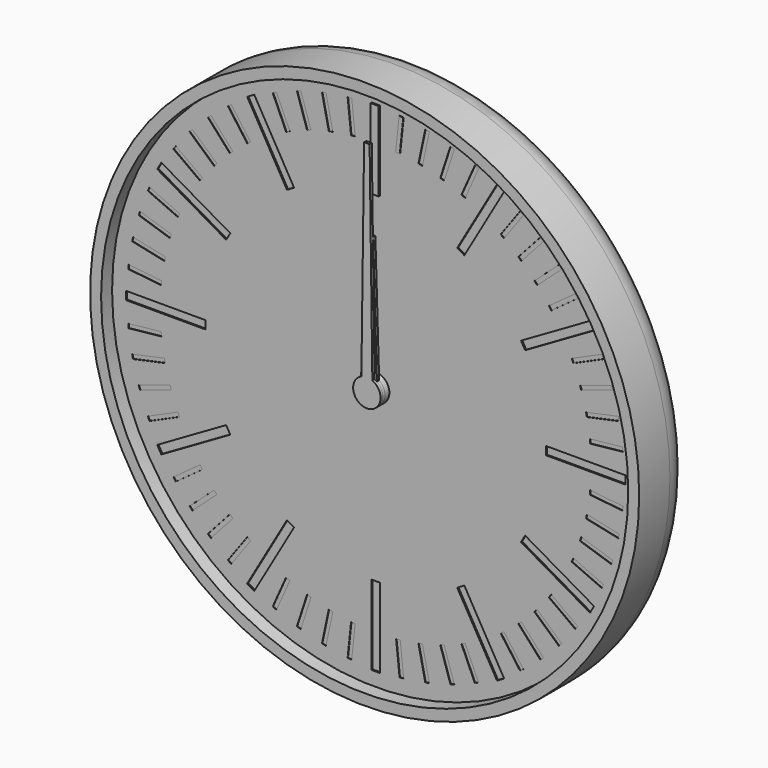
from build123d import *

# Parameters (mm, degrees)
F0_R      = 100
F1_DEPTH  = 24
F2_R      = 10
F3_T      = -4
F4_R      = 5
F4_R_2    = 3
F5_DEPTH  = 2
F6_DEPTH  = 19
F7_DEPTH  = 8
F9_DEPTH  = 4
F11_DEPTH = 4
F12_R     = 5
F12_R_2   = 3
F13_DEPTH = 2
F14_R     = 3
F15_DEPTH = 4
F17_DEPTH = 4
F18_R     = 3
F19_DEPTH = 2
F20_R     = 98
F20_R_2   = 5
F21_DEPTH = 1
F23_R     = 5
F23_R_2   = 3
F24_DEPTH = 2
F25_W     = 3
F25_H     = 29
F25_W_2   = 29
F25_H_2   = 3
F26_DEPTH = 0.5
F27_W     = 1.5
F27_H     = 12
F27_W_2   = 12
F27_H_2   = 1.5
F28_DEPTH = 0.2
F29_DEPTH = 1
F30_DEPTH = 0.4
F31_R     = 5
F31_R_2   = 3
F32_DEPTH = 5
F33_R     = 3
F34_DEPTH = 1
F36_DEPTH = 1


with BuildPart() as f1:
    # F0 (on Front) → F1 (new body)
    with BuildSketch(Plane.XZ):
        Circle(F0_R)
    extrude(amount=F1_DEPTH)

    # F2
    f2_edges = [f1.edges().sort_by_distance(p)[0] for p in [
        (-100, 0, 0),
    ]]
    fillet(f2_edges, radius=F2_R)

    # F3
    f3_openings = [f1.faces().sort_by_distance(p)[0] for p in [
        (0, -24, 0),
    ]]
    offset(amount=F3_T, openings=f3_openings)

    # F4 (on face) → F5 (join)
    with BuildSketch(Plane.XZ.offset(4)):
        Circle(F4_R)
        Circle(F4_R_2, mode=Mode.SUBTRACT)
        with Locations((40, 0)):
            Circle(F4_R)
        with Locations((40, 0)):
            Circle(F4_R_2, mode=Mode.SUBTRACT)
    extrude(amount=F5_DEPTH)


with BuildPart() as f6:
    # F6 (new): a face of the model
    f6_faces = [f1.part.faces().sort_by_distance(p)[0] for p in [
        (0, -4, 0),
    ]]
    extrude(f6_faces, amount=F6_DEPTH)

    # F8 (on face) → F9 (join)
    with BuildSketch(Plane.XZ.offset(6)):
        with BuildLine():
            ThreePointArc((9.2729637667, -1.3794085621), (9.3494561423, -0.6915886375), (9.375, 0))
            ThreePointArc((9.375, 0), (9.3494561423, 0.6915886375), (9.2729637667, 1.3794085621))
            ThreePointArc((9.2729637667, 1.3794085621), (8.9161548403, 2.8970343223), (8.3127812852, 4.3345463782))
            ThreePointArc((8.3127812852, 4.3345463782), (7.5845343223, 5.5104867402), (6.6911892658, 6.566476316))
            ThreePointArc((6.6911892658, 6.566476316), (5.5104867402, 7.5845343223), (4.1773988938, 8.3928519278))
            ThreePointArc((4.1773988938, 8.3928519278), (2.8970343223, 8.9161548403), (1.5536078905, 9.2453733036))
            ThreePointArc((1.5536078905, 9.2453733036), (0, 9.375), (-1.5536078905, 9.2453733036))
            ThreePointArc((-1.5536078905, 9.2453733036), (-2.8970343223, 8.9161548403), (-4.1773988938, 8.3928519278))
            ThreePointArc((-4.1773988938, 8.3928519278), (-5.5104867402, 7.5845343223), (-6.6911892658, 6.566476316))
            ThreePointArc((-6.6911892658, 6.566476316), (-7.5845343223, 5.5104867402), (-8.3127812852, 4.3345463782))
            ThreePointArc((-8.3127812852, 4.3345463782), (-8.9161548403, 2.8970343223), (-9.2729637667, 1.3794085621))
            ThreePointArc((-9.2729637667, 1.3794085621), (-9.375, 0), (-9.2729637667, -1.3794085621))
            ThreePointArc((-9.2729637667, -1.3794085621), (-8.9161548403, -2.8970343223), (-8.3127812852, -4.3345463782))
            ThreePointArc((-8.3127812852, -4.3345463782), (-7.5845343223, -5.5104867402), (-6.6911892658, -6.566476316))
            ThreePointArc((-6.6911892658, -6.566476316), (-5.5104867402, -7.5845343223), (-4.1773988938, -8.3928519278))
            ThreePointArc((-4.1773988938, -8.3928519278), (-2.8970343223, -8.9161548403), (-1.5536078905, -9.2453733036))
            ThreePointArc((-1.5536078905, -9.2453733036), (0, -9.375), (1.5536078905, -9.2453733036))
            ThreePointArc((1.5536078905, -9.2453733036), (2.8970343223, -8.9161548403), (4.1773988938, -8.3928519278))
            ThreePointArc((4.1773988938, -8.3928519278), (5.5104867402, -7.5845343223), (6.6911892658, -6.566476316))
            ThreePointArc((6.6911892658, -6.566476316), (7.5845343223, -5.5104867402), (8.3127812852, -4.3345463782))
            ThreePointArc((8.3127812852, -4.3345463782), (8.9161548403, -2.8970343223), (9.2729637667, -1.3794085621))
        make_face()
        with BuildLine():
            ThreePointArc((8.3127812852, 4.3345463782), (8.9161548403, 2.8970343223), (9.2729637667, 1.3794085621))
            Line((9.2729637667, 1.3794085621), (11.1823199426, 2.3946312492))
            Line((11.1823199426, 2.3946312492), (10.8182678729, 3.515068311))
            Line((10.8182678729, 3.515068311), (10.4542158031, 4.6355053728))
            Line((10.4542158031, 4.6355053728), (8.3127812852, 4.3345463782))
        make_face()
        with BuildLine():
            Line((11.1823199426, -2.3946312492), (9.2729637667, -1.3794085621))
            ThreePointArc((9.2729637667, -1.3794085621), (8.9161548403, -2.8970343223), (8.3127812852, -4.3345463782))
            Line((8.3127812852, -4.3345463782), (10.4542158031, -4.6355053728))
            Line((10.4542158031, -4.6355053728), (10.8182678729, -3.515068311))
            Line((10.8182678729, -3.515068311), (11.1823199426, -2.3946312492))
        make_face()
        with BuildLine():
            ThreePointArc((4.1773988938, 8.3928519278), (5.5104867402, 7.5845343223), (6.6911892658, 6.566476316))
            Line((6.6911892658, 6.566476316), (7.6391579371, 8.5101001246))
            Line((7.6391579371, 8.5101001246), (6.6860572448, 9.202568311))
            Line((6.6860572448, 9.202568311), (5.7329565525, 9.8950364974))
            Line((5.7329565525, 9.8950364974), (4.1773988938, 8.3928519278))
        make_face()
        with BuildLine():
            Line((7.6391579371, -8.5101001246), (6.6911892658, -6.566476316))
            ThreePointArc((6.6911892658, -6.566476316), (5.5104867402, -7.5845343223), (4.1773988938, -8.3928519278))
            Line((4.1773988938, -8.3928519278), (5.7329565525, -9.8950364974))
            Line((5.7329565525, -9.8950364974), (6.6860572448, -9.202568311))
            Line((6.6860572448, -9.202568311), (7.6391579371, -8.5101001246))
        make_face()
        with BuildLine():
            ThreePointArc((-1.5536078905, 9.2453733036), (0, 9.375), (1.5536078905, 9.2453733036))
            Line((1.5536078905, 9.2453733036), (1.1780972451, 11.375))
            Line((1.1780972451, 11.375), (0, 11.375))
            Line((0, 11.375), (-1.1780972451, 11.375))
            Line((-1.1780972451, 11.375), (-1.5536078905, 9.2453733036))
        make_face()
        with BuildLine():
            Line((1.1780972451, -11.375), (1.5536078905, -9.2453733036))
            ThreePointArc((1.5536078905, -9.2453733036), (0, -9.375), (-1.5536078905, -9.2453733036))
            Line((-1.5536078905, -9.2453733036), (-1.1780972451, -11.375))
            Line((-1.1780972451, -11.375), (0, -11.375))
            Line((0, -11.375), (1.1780972451, -11.375))
        make_face()
        with BuildLine():
            ThreePointArc((-6.6911892658, 6.566476316), (-5.5104867402, 7.5845343223), (-4.1773988938, 8.3928519278))
            Line((-4.1773988938, 8.3928519278), (-5.7329565525, 9.8950364974))
            Line((-5.7329565525, 9.8950364974), (-6.6860572448, 9.202568311))
            Line((-6.6860572448, 9.202568311), (-7.6391579371, 8.5101001246))
            Line((-7.6391579371, 8.5101001246), (-6.6911892658, 6.566476316))
        make_face()
        with BuildLine():
            Line((-5.7329565525, -9.8950364974), (-4.1773988938, -8.3928519278))
            ThreePointArc((-4.1773988938, -8.3928519278), (-5.5104867402, -7.5845343223), (-6.6911892658, -6.566476316))
            Line((-6.6911892658, -6.566476316), (-7.6391579371, -8.5101001246))
            Line((-7.6391579371, -8.5101001246), (-6.6860572448, -9.202568311))
            Line((-6.6860572448, -9.202568311), (-5.7329565525, -9.8950364974))
        make_face()
        with BuildLine():
            ThreePointArc((-9.2729637667, 1.3794085621), (-8.9161548403, 2.8970343223), (-8.3127812852, 4.3345463782))
            Line((-8.3127812852, 4.3345463782), (-10.4542158031, 4.6355053728))
            Line((-10.4542158031, 4.6355053728), (-10.8182678729, 3.515068311))
            Line((-10.8182678729, 3.515068311), (-11.1823199426, 2.3946312492))
            Line((-11.1823199426, 2.3946312492), (-9.2729637667, 1.3794085621))
        make_face()
        with BuildLine():
            Line((-10.4542158031, -4.6355053728), (-8.3127812852, -4.3345463782))
            ThreePointArc((-8.3127812852, -4.3345463782), (-8.9161548403, -2.8970343223), (-9.2729637667, -1.3794085621))
            Line((-9.2729637667, -1.3794085621), (-11.1823199426, -2.3946312492))
            Line((-11.1823199426, -2.3946312492), (-10.8182678729, -3.515068311))
            Line((-10.8182678729, -3.515068311), (-10.4542158031, -4.6355053728))
        make_face()
    extrude(amount=F9_DEPTH)

    # F35 (on face) → F36 (join)
    with BuildSketch(Plane.XZ.offset(23)):
        with BuildLine():
            ThreePointArc((-2, 4.582575695), (-2.7386127875, -4.1833001327), (5, 0))
            ThreePointArc((5, 0), (4.1833001327, 2.7386127875), (2, 4.582575695))
            ThreePointArc((2, 4.582575695), (0, 5), (-2, 4.582575695))
        make_face()
        with BuildLine():
            ThreePointArc((-2, 4.582575695), (0, 5), (2, 4.582575695))
            Line((2, 4.582575695), (1, 80))
            Line((1, 80), (0, 80))
            Line((0, 80), (-1, 80))
            Line((-1, 80), (-2, 4.582575695))
        make_face()
    extrude(amount=-F36_DEPTH)


with BuildPart() as f7:
    # F7 (new): a face of the model
    f7_faces = [f1.part.faces().sort_by_distance(p)[0] for p in [
        (40, -4, 0),
    ]]
    extrude(f7_faces, amount=F7_DEPTH)

    # F10 (on face) → F11 (join)
    with BuildSketch(Plane.XZ.offset(6)):
        with BuildLine():
            ThreePointArc((68.0829066802, -1.5381733945), (68.1144747006, -0.7693746225), (68.125, 0))
            ThreePointArc((68.125, 0), (68.1144747006, 0.7693746225), (68.0829066802, 1.5381733945))
            ThreePointArc((68.0829066802, 1.5381733945), (67.9709283072, 2.9398630294), (67.7890320221, 4.3342039956))
            ThreePointArc((67.7890320221, 4.3342039956), (67.5104012706, 5.8475163042), (67.1494235596, 7.3433252263))
            ThreePointArc((67.1494235596, 7.3433252263), (66.7484645208, 8.6911029668), (66.280643318, 10.0171558733))
            ThreePointArc((66.280643318, 10.0171558733), (65.6934659962, 11.4394680865), (65.0293803521, 12.8275385085))
            ThreePointArc((65.0293803521, 12.8275385085), (64.3569644814, 14.0625), (63.6236643925, 15.2623099717))
            ThreePointArc((63.6236643925, 15.2623099717), (62.7536029668, 16.5314602207), (61.815433119, 17.7511268046))
            ThreePointArc((61.815433119, 17.7511268046), (60.9009482166, 18.8192983038), (59.934217974, 19.8404278876))
            ThreePointArc((59.934217974, 19.8404278876), (58.8192983038, 20.9009482166), (57.6480467764, 21.8989056799))
            ThreePointArc((57.6480467764, 21.8989056799), (56.5314602207, 22.7536029668), (55.3735505752, 23.5514238999))
            ThreePointArc((55.3735505752, 23.5514238999), (54.0625, 24.3569644814), (52.709356105, 25.0895972944))
            ThreePointArc((52.709356105, 25.0895972944), (51.4394680865, 25.6934659962), (50.1409852457, 26.2331096755))
            ThreePointArc((50.1409852457, 26.2331096755), (48.6911029668, 26.7484645208), (47.2152055856, 27.1837531139))
            ThreePointArc((47.2152055856, 27.1837531139), (45.8475163042, 27.5104012706), (44.4652101991, 27.7682826779))
            ThreePointArc((44.4652101991, 27.7682826779), (42.9398630294, 27.9709283072), (41.4057159597, 28.0898484802))
            ThreePointArc((41.4057159597, 28.0898484802), (40, 28.125), (38.5942840403, 28.0898484802))
            ThreePointArc((38.5942840403, 28.0898484802), (37.0601369706, 27.9709283072), (35.5347898009, 27.7682826779))
            ThreePointArc((35.5347898009, 27.7682826779), (34.1524836958, 27.5104012706), (32.7847944144, 27.1837531139))
            ThreePointArc((32.7847944144, 27.1837531139), (31.3088970332, 26.7484645208), (29.8590147543, 26.2331096755))
            ThreePointArc((29.8590147543, 26.2331096755), (28.5605319135, 25.6934659962), (27.290643895, 25.0895972944))
            ThreePointArc((27.290643895, 25.0895972944), (25.9375, 24.3569644814), (24.6264494248, 23.5514238999))
            ThreePointArc((24.6264494248, 23.5514238999), (23.4685397793, 22.7536029668), (22.3519532236, 21.8989056799))
            ThreePointArc((22.3519532236, 21.8989056799), (21.1807016962, 20.9009482166), (20.065782026, 19.8404278876))
            ThreePointArc((20.065782026, 19.8404278876), (19.0990517834, 18.8192983038), (18.184566881, 17.7511268046))
            ThreePointArc((18.184566881, 17.7511268046), (17.2463970332, 16.5314602207), (16.3763356075, 15.2623099717))
            ThreePointArc((16.3763356075, 15.2623099717), (15.6430355186, 14.0625), (14.9706196479, 12.8275385085))
            ThreePointArc((14.9706196479, 12.8275385085), (14.3065340038, 11.4394680865), (13.719356682, 10.0171558733))
            ThreePointArc((13.719356682, 10.0171558733), (13.2515354792, 8.6911029668), (12.8505764404, 7.3433252263))
            ThreePointArc((12.8505764404, 7.3433252263), (12.4895987294, 5.8475163042), (12.2109679779, 4.3342039956))
            ThreePointArc((12.2109679779, 4.3342039956), (12.0290716928, 2.9398630294), (11.9170933198, 1.5381733945))
            ThreePointArc((11.9170933198, 1.5381733945), (11.875, 0), (11.9170933198, -1.5381733945))
            ThreePointArc((11.9170933198, -1.5381733945), (12.0290716928, -2.9398630294), (12.2109679779, -4.3342039956))
            ThreePointArc((12.2109679779, -4.3342039956), (12.4895987294, -5.8475163042), (12.8505764404, -7.3433252263))
            ThreePointArc((12.8505764404, -7.3433252263), (13.2515354792, -8.6911029668), (13.719356682, -10.0171558733))
            ThreePointArc((13.719356682, -10.0171558733), (14.3065340038, -11.4394680865), (14.9706196479, -12.8275385085))
            ThreePointArc((14.9706196479, -12.8275385085), (15.6430355186, -14.0625), (16.3763356075, -15.2623099717))
            ThreePointArc((16.3763356075, -15.2623099717), (17.2463970332, -16.5314602207), (18.184566881, -17.7511268046))
            ThreePointArc((18.184566881, -17.7511268046), (19.0990517834, -18.8192983038), (20.065782026, -19.8404278876))
            ThreePointArc((20.065782026, -19.8404278876), (21.1807016962, -20.9009482166), (22.3519532236, -21.8989056799))
            ThreePointArc((22.3519532236, -21.8989056799), (23.4685397793, -22.7536029668), (24.6264494248, -23.5514238999))
            ThreePointArc((24.6264494248, -23.5514238999), (25.9375, -24.3569644814), (27.290643895, -25.0895972944))
            ThreePointArc((27.290643895, -25.0895972944), (28.5605319135, -25.6934659962), (29.8590147543, -26.2331096755))
            ThreePointArc((29.8590147543, -26.2331096755), (31.3088970332, -26.7484645208), (32.7847944144, -27.1837531139))
            ThreePointArc((32.7847944144, -27.1837531139), (34.1524836958, -27.5104012706), (35.5347898009, -27.7682826779))
            ThreePointArc((35.5347898009, -27.7682826779), (37.0601369706, -27.9709283072), (38.5942840403, -28.0898484802))
            ThreePointArc((38.5942840403, -28.0898484802), (40, -28.125), (41.4057159597, -28.0898484802))
            ThreePointArc((41.4057159597, -28.0898484802), (42.9398630294, -27.9709283072), (44.4652101991, -27.7682826779))
            ThreePointArc((44.4652101991, -27.7682826779), (45.8475163042, -27.5104012706), (47.2152055856, -27.1837531139))
            ThreePointArc((47.2152055856, -27.1837531139), (48.6911029668, -26.7484645208), (50.1409852457, -26.2331096755))
            ThreePointArc((50.1409852457, -26.2331096755), (51.4394680865, -25.6934659962), (52.709356105, -25.0895972944))
            ThreePointArc((52.709356105, -25.0895972944), (54.0625, -24.3569644814), (55.3735505752, -23.5514238999))
            ThreePointArc((55.3735505752, -23.5514238999), (56.5314602207, -22.7536029668), (57.6480467764, -21.8989056799))
            ThreePointArc((57.6480467764, -21.8989056799), (58.8192983038, -20.9009482166), (59.934217974, -19.8404278876))
            ThreePointArc((59.934217974, -19.8404278876), (60.9009482166, -18.8192983038), (61.815433119, -17.7511268046))
            ThreePointArc((61.815433119, -17.7511268046), (62.7536029668, -16.5314602207), (63.6236643925, -15.2623099717))
            ThreePointArc((63.6236643925, -15.2623099717), (64.3569644814, -14.0625), (65.0293803521, -12.8275385085))
            ThreePointArc((65.0293803521, -12.8275385085), (65.6934659962, -11.4394680865), (66.280643318, -10.0171558733))
            ThreePointArc((66.280643318, -10.0171558733), (66.7484645208, -8.6911029668), (67.1494235596, -7.3433252263))
            ThreePointArc((67.1494235596, -7.3433252263), (67.5104012706, -5.8475163042), (67.7890320221, -4.3342039956))
            ThreePointArc((67.7890320221, -4.3342039956), (67.9709283072, -2.9398630294), (68.0829066802, -1.5381733945))
        make_face()
        with BuildLine():
            ThreePointArc((68.0829066802, 1.5381733945), (68.1144747006, 0.7693746225), (68.125, 0))
            ThreePointArc((68.125, 0), (68.1144747006, -0.7693746225), (68.0829066802, -1.5381733945))
            Line((68.0829066802, -1.5381733945), (70.125, -1.1780972451))
            Line((70.125, -1.1780972451), (70.125, 0))
            Line((70.125, 0), (70.125, 1.1780972451))
            Line((70.125, 1.1780972451), (68.0829066802, 1.5381733945))
        make_face()
        with BuildLine():
            ThreePointArc((67.1494235596, 7.3433252263), (67.5104012706, 5.8475163042), (67.7890320221, 4.3342039956))
            Line((67.7890320221, 4.3342039956), (69.7116366623, 5.1109866922))
            Line((69.7116366623, 5.1109866922), (69.4666964721, 6.2633396859))
            Line((69.4666964721, 6.2633396859), (69.2217562819, 7.4156926796))
            Line((69.2217562819, 7.4156926796), (67.1494235596, 7.3433252263))
        make_face()
        with BuildLine():
            Line((69.7116366623, -5.1109866922), (67.7890320221, -4.3342039956))
            ThreePointArc((67.7890320221, -4.3342039956), (67.5104012706, -5.8475163042), (67.1494235596, -7.3433252263))
            Line((67.1494235596, -7.3433252263), (69.2217562819, -7.4156926796))
            Line((69.2217562819, -7.4156926796), (69.4666964721, -6.2633396859))
            Line((69.4666964721, -6.2633396859), (69.7116366623, -5.1109866922))
        make_face()
        with BuildLine():
            ThreePointArc((65.0293803521, 12.8275385085), (65.6934659962, 11.4394680865), (66.280643318, 10.0171558733))
            Line((66.280643318, 10.0171558733), (67.9997322302, 11.1766959857))
            Line((67.9997322302, 11.1766959857), (67.5205569115, 12.2529413727))
            Line((67.5205569115, 12.2529413727), (67.0413815928, 13.3291867596))
            Line((67.0413815928, 13.3291867596), (65.0293803521, 12.8275385085))
        make_face()
        with BuildLine():
            Line((67.9997322302, -11.1766959857), (66.280643318, -10.0171558733))
            ThreePointArc((66.280643318, -10.0171558733), (65.6934659962, -11.4394680865), (65.0293803521, -12.8275385085))
            Line((65.0293803521, -12.8275385085), (67.0413815928, -13.3291867596))
            Line((67.0413815928, -13.3291867596), (67.5205569115, -12.2529413727))
            Line((67.5205569115, -12.2529413727), (67.9997322302, -11.1766959857))
        make_face()
        with BuildLine():
            ThreePointArc((61.815433119, 17.7511268046), (62.7536029668, 16.5314602207), (63.6236643925, 15.2623099717))
            Line((63.6236643925, 15.2623099717), (65.064105142, 16.753930033))
            Line((65.064105142, 16.753930033), (64.3716369555, 17.7070307253))
            Line((64.3716369555, 17.7070307253), (63.6791687691, 18.6601314176))
            Line((63.6791687691, 18.6601314176), (61.815433119, 17.7511268046))
        make_face()
        with BuildLine():
            Line((65.064105142, -16.753930033), (63.6236643925, -15.2623099717))
            ThreePointArc((63.6236643925, -15.2623099717), (62.7536029668, -16.5314602207), (61.815433119, -17.7511268046))
            Line((61.815433119, -17.7511268046), (63.6791687691, -18.6601314176))
            Line((63.6791687691, -18.6601314176), (64.3716369555, -17.7070307253))
            Line((64.3716369555, -17.7070307253), (65.064105142, -16.753930033))
        make_face()
        with BuildLine():
            ThreePointArc((57.6480467764, 21.8989056799), (58.8192983038, 20.9009482166), (59.934217974, 19.8404278876))
            Line((59.934217974, 19.8404278876), (61.0330563882, 21.5989369435))
            Line((61.0330563882, 21.5989369435), (60.1575595166, 22.3872378675))
            Line((60.1575595166, 22.3872378675), (59.282062645, 23.1755387915))
            Line((59.282062645, 23.1755387915), (57.6480467764, 21.8989056799))
        make_face()
        with BuildLine():
            Line((61.0330563882, -21.5989369435), (59.934217974, -19.8404278876))
            ThreePointArc((59.934217974, -19.8404278876), (58.8192983038, -20.9009482166), (57.6480467764, -21.8989056799))
            Line((57.6480467764, -21.8989056799), (59.282062645, -23.1755387915))
            Line((59.282062645, -23.1755387915), (60.1575595166, -22.3872378675))
            Line((60.1575595166, -22.3872378675), (61.0330563882, -21.5989369435))
        make_face()
        with BuildLine():
            ThreePointArc((52.709356105, 25.0895972944), (54.0625, 24.3569644814), (55.3735505752, 23.5514238999))
            Line((55.3735505752, 23.5514238999), (56.0827621424, 25.4999666665))
            Line((56.0827621424, 25.4999666665), (55.0625, 26.089015289))
            Line((55.0625, 26.089015289), (54.0422378576, 26.6780639116))
            Line((54.0422378576, 26.6780639116), (52.709356105, 25.0895972944))
        make_face()
        with BuildLine():
            Line((56.0827621424, -25.4999666665), (55.3735505752, -23.5514238999))
            ThreePointArc((55.3735505752, -23.5514238999), (54.0625, -24.3569644814), (52.709356105, -25.0895972944))
            Line((52.709356105, -25.0895972944), (54.0422378576, -26.6780639116))
            Line((54.0422378576, -26.6780639116), (55.0625, -26.089015289))
            Line((55.0625, -26.089015289), (56.0827621424, -25.4999666665))
        make_face()
        with BuildLine():
            ThreePointArc((47.2152055856, 27.1837531139), (48.6911029668, 26.7484645208), (50.1409852457, 26.2331096755))
            Line((50.1409852457, 26.2331096755), (50.4295740173, 28.2865254836))
            Line((50.4295740173, 28.2865254836), (49.3091369555, 28.6505775534))
            Line((49.3091369555, 28.6505775534), (48.1886998938, 29.0146296232))
            Line((48.1886998938, 29.0146296232), (47.2152055856, 27.1837531139))
        make_face()
        with BuildLine():
            Line((50.4295740173, -28.2865254836), (50.1409852457, -26.2331096755))
            ThreePointArc((50.1409852457, -26.2331096755), (48.6911029668, -26.7484645208), (47.2152055856, -27.1837531139))
            Line((47.2152055856, -27.1837531139), (48.1886998938, -29.0146296232))
            Line((48.1886998938, -29.0146296232), (49.3091369555, -28.6505775534))
            Line((49.3091369555, -28.6505775534), (50.4295740173, -28.2865254836))
        make_face()
        with BuildLine():
            ThreePointArc((41.4057159597, 28.0898484802), (42.9398630294, 27.9709283072), (44.4652101991, 27.7682826779))
            Line((44.4652101991, 27.7682826779), (44.3205634611, 29.8368274034))
            Line((44.3205634611, 29.8368274034), (43.1489199559, 29.959972098))
            Line((43.1489199559, 29.959972098), (41.9772764508, 30.0831167926))
            Line((41.9772764508, 30.0831167926), (41.4057159597, 28.0898484802))
        make_face()
        with BuildLine():
            Line((44.3205634611, -29.8368274034), (44.4652101991, -27.7682826779))
            ThreePointArc((44.4652101991, -27.7682826779), (42.9398630294, -27.9709283072), (41.4057159597, -28.0898484802))
            Line((41.4057159597, -28.0898484802), (41.9772764508, -30.0831167926))
            Line((41.9772764508, -30.0831167926), (43.1489199559, -29.959972098))
            Line((43.1489199559, -29.959972098), (44.3205634611, -29.8368274034))
        make_face()
        with BuildLine():
            ThreePointArc((35.5347898009, 27.7682826779), (37.0601369706, 27.9709283072), (38.5942840403, 28.0898484802))
            Line((38.5942840403, 28.0898484802), (38.0227235492, 30.0831167926))
            Line((38.0227235492, 30.0831167926), (36.8510800441, 29.959972098))
            Line((36.8510800441, 29.959972098), (35.6794365389, 29.8368274034))
            Line((35.6794365389, 29.8368274034), (35.5347898009, 27.7682826779))
        make_face()
        with BuildLine():
            Line((38.0227235492, -30.0831167926), (38.5942840403, -28.0898484802))
            ThreePointArc((38.5942840403, -28.0898484802), (37.0601369706, -27.9709283072), (35.5347898009, -27.7682826779))
            Line((35.5347898009, -27.7682826779), (35.6794365389, -29.8368274034))
            Line((35.6794365389, -29.8368274034), (36.8510800441, -29.959972098))
            Line((36.8510800441, -29.959972098), (38.0227235492, -30.0831167926))
        make_face()
        with BuildLine():
            ThreePointArc((29.8590147543, 26.2331096755), (31.3088970332, 26.7484645208), (32.7847944144, 27.1837531139))
            Line((32.7847944144, 27.1837531139), (31.8113001062, 29.0146296232))
            Line((31.8113001062, 29.0146296232), (30.6908630445, 28.6505775534))
            Line((30.6908630445, 28.6505775534), (29.5704259827, 28.2865254836))
            Line((29.5704259827, 28.2865254836), (29.8590147543, 26.2331096755))
        make_face()
        with BuildLine():
            Line((31.8113001062, -29.0146296232), (32.7847944144, -27.1837531139))
            ThreePointArc((32.7847944144, -27.1837531139), (31.3088970332, -26.7484645208), (29.8590147543, -26.2331096755))
            Line((29.8590147543, -26.2331096755), (29.5704259827, -28.2865254836))
            Line((29.5704259827, -28.2865254836), (30.6908630445, -28.6505775534))
            Line((30.6908630445, -28.6505775534), (31.8113001062, -29.0146296232))
        make_face()
        with BuildLine():
            ThreePointArc((24.6264494248, 23.5514238999), (25.9375, 24.3569644814), (27.290643895, 25.0895972944))
            Line((27.290643895, 25.0895972944), (25.9577621424, 26.6780639116))
            Line((25.9577621424, 26.6780639116), (24.9375, 26.089015289))
            Line((24.9375, 26.089015289), (23.9172378576, 25.4999666665))
            Line((23.9172378576, 25.4999666665), (24.6264494248, 23.5514238999))
        make_face()
        with BuildLine():
            Line((25.9577621424, -26.6780639116), (27.290643895, -25.0895972944))
            ThreePointArc((27.290643895, -25.0895972944), (25.9375, -24.3569644814), (24.6264494248, -23.5514238999))
            Line((24.6264494248, -23.5514238999), (23.9172378576, -25.4999666665))
            Line((23.9172378576, -25.4999666665), (24.9375, -26.089015289))
            Line((24.9375, -26.089015289), (25.9577621424, -26.6780639116))
        make_face()
        with BuildLine():
            ThreePointArc((20.065782026, 19.8404278876), (21.1807016962, 20.9009482166), (22.3519532236, 21.8989056799))
            Line((22.3519532236, 21.8989056799), (20.717937355, 23.1755387915))
            Line((20.717937355, 23.1755387915), (19.8424404834, 22.3872378675))
            Line((19.8424404834, 22.3872378675), (18.9669436118, 21.5989369435))
            Line((18.9669436118, 21.5989369435), (20.065782026, 19.8404278876))
        make_face()
        with BuildLine():
            Line((20.717937355, -23.1755387915), (22.3519532236, -21.8989056799))
            ThreePointArc((22.3519532236, -21.8989056799), (21.1807016962, -20.9009482166), (20.065782026, -19.8404278876))
            Line((20.065782026, -19.8404278876), (18.9669436118, -21.5989369435))
            Line((18.9669436118, -21.5989369435), (19.8424404834, -22.3872378675))
            Line((19.8424404834, -22.3872378675), (20.717937355, -23.1755387915))
        make_face()
        with BuildLine():
            ThreePointArc((16.3763356075, 15.2623099717), (17.2463970332, 16.5314602207), (18.184566881, 17.7511268046))
            Line((18.184566881, 17.7511268046), (16.3208312309, 18.6601314176))
            Line((16.3208312309, 18.6601314176), (15.6283630445, 17.7070307253))
            Line((15.6283630445, 17.7070307253), (14.935894858, 16.753930033))
            Line((14.935894858, 16.753930033), (16.3763356075, 15.2623099717))
        make_face()
        with BuildLine():
            Line((16.3208312309, -18.6601314176), (18.184566881, -17.7511268046))
            ThreePointArc((18.184566881, -17.7511268046), (17.2463970332, -16.5314602207), (16.3763356075, -15.2623099717))
            Line((16.3763356075, -15.2623099717), (14.935894858, -16.753930033))
            Line((14.935894858, -16.753930033), (15.6283630445, -17.7070307253))
            Line((15.6283630445, -17.7070307253), (16.3208312309, -18.6601314176))
        make_face()
        with BuildLine():
            ThreePointArc((13.719356682, 10.0171558733), (14.3065340038, 11.4394680865), (14.9706196479, 12.8275385085))
            Line((14.9706196479, 12.8275385085), (12.9586184072, 13.3291867596))
            Line((12.9586184072, 13.3291867596), (12.4794430885, 12.2529413727))
            Line((12.4794430885, 12.2529413727), (12.0002677698, 11.1766959857))
            Line((12.0002677698, 11.1766959857), (13.719356682, 10.0171558733))
        make_face()
        with BuildLine():
            Line((12.9586184072, -13.3291867596), (14.9706196479, -12.8275385085))
            ThreePointArc((14.9706196479, -12.8275385085), (14.3065340038, -11.4394680865), (13.719356682, -10.0171558733))
            Line((13.719356682, -10.0171558733), (12.0002677698, -11.1766959857))
            Line((12.0002677698, -11.1766959857), (12.4794430885, -12.2529413727))
            Line((12.4794430885, -12.2529413727), (12.9586184072, -13.3291867596))
        make_face()
        with BuildLine():
            ThreePointArc((12.2109679779, 4.3342039956), (12.4895987294, 5.8475163042), (12.8505764404, 7.3433252263))
            Line((12.8505764404, 7.3433252263), (10.7782437181, 7.4156926796))
            Line((10.7782437181, 7.4156926796), (10.5333035279, 6.2633396859))
            Line((10.5333035279, 6.2633396859), (10.2883633377, 5.1109866922))
            Line((10.2883633377, 5.1109866922), (12.2109679779, 4.3342039956))
        make_face()
        with BuildLine():
            Line((10.7782437181, -7.4156926796), (12.8505764404, -7.3433252263))
            ThreePointArc((12.8505764404, -7.3433252263), (12.4895987294, -5.8475163042), (12.2109679779, -4.3342039956))
            Line((12.2109679779, -4.3342039956), (10.2883633377, -5.1109866922))
            Line((10.2883633377, -5.1109866922), (10.5333035279, -6.2633396859))
            Line((10.5333035279, -6.2633396859), (10.7782437181, -7.4156926796))
        make_face()
        with BuildLine():
            ThreePointArc((11.9170933198, -1.5381733945), (11.875, 0), (11.9170933198, 1.5381733945))
            Line((11.9170933198, 1.5381733945), (9.875, 1.1780972451))
            Line((9.875, 1.1780972451), (9.875, 0))
            Line((9.875, 0), (9.875, -1.1780972451))
            Line((9.875, -1.1780972451), (11.9170933198, -1.5381733945))
        make_face()
    extrude(amount=F11_DEPTH)

    # F16 (on face) → F17 (join)
    with BuildSketch(Plane.XZ.offset(12)):
        with BuildLine():
            ThreePointArc((47.4288750323, -1.0304444454), (47.4821976298, -0.5164480894), (47.5, 0))
            ThreePointArc((47.5, 0), (47.4821976298, 0.5164480894), (47.4288750323, 1.0304444454))
            ThreePointArc((47.4288750323, 1.0304444454), (47.1329238722, 2.3176274578), (46.6157661985, 3.532936117))
            ThreePointArc((46.6157661985, 3.532936117), (46.0676274578, 4.4083893922), (45.4044061018, 5.2002302532))
            ThreePointArc((45.4044061018, 5.2002302532), (44.4083893922, 6.0676274578), (43.2756595386, 6.7468551628))
            ThreePointArc((43.2756595386, 6.7468551628), (42.3176274578, 7.1329238722), (41.3156377295, 7.3837048536))
            ThreePointArc((41.3156377295, 7.3837048536), (40, 7.5), (38.6843622705, 7.3837048536))
            ThreePointArc((38.6843622705, 7.3837048536), (37.6823725422, 7.1329238722), (36.7243404614, 6.7468551628))
            ThreePointArc((36.7243404614, 6.7468551628), (35.5916106078, 6.0676274578), (34.5955938982, 5.2002302532))
            ThreePointArc((34.5955938982, 5.2002302532), (33.9323725422, 4.4083893922), (33.3842338015, 3.532936117))
            ThreePointArc((33.3842338015, 3.532936117), (32.8670761278, 2.3176274578), (32.5711249677, 1.0304444454))
            ThreePointArc((32.5711249677, 1.0304444454), (32.5, 0), (32.5711249677, -1.0304444454))
            ThreePointArc((32.5711249677, -1.0304444454), (32.8670761278, -2.3176274578), (33.3842338015, -3.532936117))
            ThreePointArc((33.3842338015, -3.532936117), (33.9323725422, -4.4083893922), (34.5955938982, -5.2002302532))
            ThreePointArc((34.5955938982, -5.2002302532), (35.5916106078, -6.0676274578), (36.7243404614, -6.7468551628))
            ThreePointArc((36.7243404614, -6.7468551628), (37.6823725422, -7.1329238722), (38.6843622705, -7.3837048536))
            ThreePointArc((38.6843622705, -7.3837048536), (40, -7.5), (41.3156377295, -7.3837048536))
            ThreePointArc((41.3156377295, -7.3837048536), (42.3176274578, -7.1329238722), (43.2756595386, -6.7468551628))
            ThreePointArc((43.2756595386, -6.7468551628), (44.4083893922, -6.0676274578), (45.4044061018, -5.2002302532))
            ThreePointArc((45.4044061018, -5.2002302532), (46.0676274578, -4.4083893922), (46.6157661985, -3.532936117))
            ThreePointArc((46.6157661985, -3.532936117), (47.1329238722, -2.3176274578), (47.4288750323, -1.0304444454))
        make_face()
        with BuildLine():
            ThreePointArc((46.6157661985, 3.532936117), (47.1329238722, 2.3176274578), (47.4288750323, 1.0304444454))
            Line((47.4288750323, 1.0304444454), (49.3262785606, 2.0393117971))
            Line((49.3262785606, 2.0393117971), (48.743795249, 3.832011096))
            Line((48.743795249, 3.832011096), (46.6157661985, 3.532936117))
        make_face()
        with BuildLine():
            Line((49.3262785606, -2.0393117971), (47.4288750323, -1.0304444454))
            ThreePointArc((47.4288750323, -1.0304444454), (47.1329238722, -2.3176274578), (46.6157661985, -3.532936117))
            Line((46.6157661985, -3.532936117), (48.743795249, -3.832011096))
            Line((48.743795249, -3.832011096), (49.3262785606, -2.0393117971))
        make_face()
        with BuildLine():
            ThreePointArc((43.2756595386, 6.7468551628), (44.4083893922, 6.0676274578), (45.4044061018, 5.2002302532))
            Line((45.4044061018, 5.2002302532), (46.3464404506, 7.1316868974))
            Line((46.3464404506, 7.1316868974), (44.8214793429, 8.2396359957))
            Line((44.8214793429, 8.2396359957), (43.2756595386, 6.7468551628))
        make_face()
        with BuildLine():
            Line((46.3464404506, -7.1316868974), (45.4044061018, -5.2002302532))
            ThreePointArc((45.4044061018, -5.2002302532), (44.4083893922, -6.0676274578), (43.2756595386, -6.7468551628))
            Line((43.2756595386, -6.7468551628), (44.8214793429, -8.2396359957))
            Line((44.8214793429, -8.2396359957), (46.3464404506, -7.1316868974))
        make_face()
        with BuildLine():
            ThreePointArc((38.6843622705, 7.3837048536), (40, 7.5), (41.3156377295, 7.3837048536))
            Line((41.3156377295, 7.3837048536), (40.9424777961, 9.5))
            Line((40.9424777961, 9.5), (39.0575222039, 9.5))
            Line((39.0575222039, 9.5), (38.6843622705, 7.3837048536))
        make_face()
        with BuildLine():
            Line((40.9424777961, -9.5), (41.3156377295, -7.3837048536))
            ThreePointArc((41.3156377295, -7.3837048536), (40, -7.5), (38.6843622705, -7.3837048536))
            Line((38.6843622705, -7.3837048536), (39.0575222039, -9.5))
            Line((39.0575222039, -9.5), (40.9424777961, -9.5))
        make_face()
        with BuildLine():
            ThreePointArc((34.5955938982, 5.2002302532), (35.5916106078, 6.0676274578), (36.7243404614, 6.7468551628))
            Line((36.7243404614, 6.7468551628), (35.1785206571, 8.2396359957))
            Line((35.1785206571, 8.2396359957), (33.6535595494, 7.1316868974))
            Line((33.6535595494, 7.1316868974), (34.5955938982, 5.2002302532))
        make_face()
        with BuildLine():
            Line((35.1785206571, -8.2396359957), (36.7243404614, -6.7468551628))
            ThreePointArc((36.7243404614, -6.7468551628), (35.5916106078, -6.0676274578), (34.5955938982, -5.2002302532))
            Line((34.5955938982, -5.2002302532), (33.6535595494, -7.1316868974))
            Line((33.6535595494, -7.1316868974), (35.1785206571, -8.2396359957))
        make_face()
        with BuildLine():
            ThreePointArc((32.5711249677, 1.0304444454), (32.8670761278, 2.3176274578), (33.3842338015, 3.532936117))
            Line((33.3842338015, 3.532936117), (31.256204751, 3.832011096))
            Line((31.256204751, 3.832011096), (30.6737214394, 2.0393117971))
            Line((30.6737214394, 2.0393117971), (32.5711249677, 1.0304444454))
        make_face()
        with BuildLine():
            Line((31.256204751, -3.832011096), (33.3842338015, -3.532936117))
            ThreePointArc((33.3842338015, -3.532936117), (32.8670761278, -2.3176274578), (32.5711249677, -1.0304444454))
            Line((32.5711249677, -1.0304444454), (30.6737214394, -2.0393117971))
            Line((30.6737214394, -2.0393117971), (31.256204751, -3.832011096))
        make_face()
    extrude(amount=F17_DEPTH)

    # F18 (on face) → F19 (join)
    with BuildSketch(Plane.XZ.offset(16)):
        with Locations((40, 0)):
            Circle(F18_R)
    extrude(amount=F19_DEPTH)


with BuildPart() as f13:
    # F12 (on face) → F13 (new body)
    with BuildSketch(Plane.XZ.offset(10)):
        Circle(F12_R)
        Circle(F12_R_2, mode=Mode.SUBTRACT)
    extrude(amount=F13_DEPTH)

    # F14 (on face) → F15 (join)
    with BuildSketch(Plane.XZ.offset(12)):
        with BuildLine():
            ThreePointArc((29.9718156995, -1.3001014101), (29.9929530972, -0.6502034357), (30, 0))
            ThreePointArc((30, 0), (29.9929530972, 0.6502034357), (29.9718156995, 1.3001014101))
            ThreePointArc((29.9718156995, 1.3001014101), (29.907520012, 2.3537728718), (29.8061935814, 3.4045299509))
            ThreePointArc((29.8061935814, 3.4045299509), (29.6306502179, 4.6930339512), (29.3994322443, 5.9727199596))
            ThreePointArc((29.3994322443, 5.9727199596), (29.1710976119, 7.0033609157), (28.9066440563, 8.0253304855))
            ThreePointArc((28.9066440563, 8.0253304855), (28.5316954889, 9.2705098312), (28.1031371961, 10.4982703213))
            ThreePointArc((28.1031371961, 10.4982703213), (27.7163859753, 11.480502971), (27.2953170189, 12.448520749))
            ThreePointArc((27.2953170189, 12.448520749), (26.7301957257, 13.6197149922), (26.1148496411, 14.765318426))
            ThreePointArc((26.1148496411, 14.765318426), (25.5792049306, 15.6749569415), (25.0118886885, 16.5651871174))
            ThreePointArc((25.0118886885, 16.5651871174), (24.2705098312, 17.6335575688), (23.4835278178, 18.6687953878))
            ThreePointArc((23.4835278178, 18.6687953878), (22.812178968, 19.4834414499), (22.1125846489, 20.2739636023))
            ThreePointArc((22.1125846489, 20.2739636023), (21.2132034356, 21.2132034356), (20.2739636023, 22.1125846489))
            ThreePointArc((20.2739636023, 22.1125846489), (19.4834414499, 22.812178968), (18.6687953878, 23.4835278178))
            ThreePointArc((18.6687953878, 23.4835278178), (17.6335575688, 24.2705098312), (16.5651871174, 25.0118886885))
            ThreePointArc((16.5651871174, 25.0118886885), (15.6749569415, 25.5792049306), (14.765318426, 26.1148496411))
            ThreePointArc((14.765318426, 26.1148496411), (13.6197149922, 26.7301957257), (12.448520749, 27.2953170189))
            ThreePointArc((12.448520749, 27.2953170189), (11.480502971, 27.7163859753), (10.4982703213, 28.1031371961))
            ThreePointArc((10.4982703213, 28.1031371961), (9.2705098312, 28.5316954889), (8.0253304855, 28.9066440563))
            ThreePointArc((8.0253304855, 28.9066440563), (7.0033609157, 29.1710976119), (5.9727199596, 29.3994322443))
            ThreePointArc((5.9727199596, 29.3994322443), (4.6930339512, 29.6306502179), (3.4045299509, 29.8061935814))
            ThreePointArc((3.4045299509, 29.8061935814), (2.3537728718, 29.907520012), (1.3001014101, 29.9718156995))
            ThreePointArc((1.3001014101, 29.9718156995), (0, 30), (-1.3001014101, 29.9718156995))
            ThreePointArc((-1.3001014101, 29.9718156995), (-2.3537728718, 29.907520012), (-3.4045299509, 29.8061935814))
            ThreePointArc((-3.4045299509, 29.8061935814), (-4.6930339512, 29.6306502179), (-5.9727199596, 29.3994322443))
            ThreePointArc((-5.9727199596, 29.3994322443), (-7.0033609157, 29.1710976119), (-8.0253304855, 28.9066440563))
            ThreePointArc((-8.0253304855, 28.9066440563), (-9.2705098312, 28.5316954889), (-10.4982703213, 28.1031371961))
            ThreePointArc((-10.4982703213, 28.1031371961), (-11.480502971, 27.7163859753), (-12.448520749, 27.2953170189))
            ThreePointArc((-12.448520749, 27.2953170189), (-13.6197149922, 26.7301957257), (-14.765318426, 26.1148496411))
            ThreePointArc((-14.765318426, 26.1148496411), (-15.6749569415, 25.5792049306), (-16.5651871174, 25.0118886885))
            ThreePointArc((-16.5651871174, 25.0118886885), (-17.6335575688, 24.2705098312), (-18.6687953878, 23.4835278178))
            ThreePointArc((-18.6687953878, 23.4835278178), (-19.4834414499, 22.812178968), (-20.2739636023, 22.1125846489))
            ThreePointArc((-20.2739636023, 22.1125846489), (-21.2132034356, 21.2132034356), (-22.1125846489, 20.2739636023))
            ThreePointArc((-22.1125846489, 20.2739636023), (-22.812178968, 19.4834414499), (-23.4835278178, 18.6687953878))
            ThreePointArc((-23.4835278178, 18.6687953878), (-24.2705098312, 17.6335575688), (-25.0118886885, 16.5651871174))
            ThreePointArc((-25.0118886885, 16.5651871174), (-25.5792049306, 15.6749569415), (-26.1148496411, 14.765318426))
            ThreePointArc((-26.1148496411, 14.765318426), (-26.7301957257, 13.6197149922), (-27.2953170189, 12.448520749))
            ThreePointArc((-27.2953170189, 12.448520749), (-27.7163859753, 11.480502971), (-28.1031371961, 10.4982703213))
            ThreePointArc((-28.1031371961, 10.4982703213), (-28.5316954889, 9.2705098312), (-28.9066440563, 8.0253304855))
            ThreePointArc((-28.9066440563, 8.0253304855), (-29.1710976119, 7.0033609157), (-29.3994322443, 5.9727199596))
            ThreePointArc((-29.3994322443, 5.9727199596), (-29.6306502179, 4.6930339512), (-29.8061935814, 3.4045299509))
            ThreePointArc((-29.8061935814, 3.4045299509), (-29.907520012, 2.3537728718), (-29.9718156995, 1.3001014101))
            ThreePointArc((-29.9718156995, 1.3001014101), (-30, 0), (-29.9718156995, -1.3001014101))
            ThreePointArc((-29.9718156995, -1.3001014101), (-29.907520012, -2.3537728718), (-29.8061935814, -3.4045299509))
            ThreePointArc((-29.8061935814, -3.4045299509), (-29.6306502179, -4.6930339512), (-29.3994322443, -5.9727199596))
            ThreePointArc((-29.3994322443, -5.9727199596), (-29.1710976119, -7.0033609157), (-28.9066440563, -8.0253304855))
            ThreePointArc((-28.9066440563, -8.0253304855), (-28.5316954889, -9.2705098312), (-28.1031371961, -10.4982703213))
            ThreePointArc((-28.1031371961, -10.4982703213), (-27.7163859753, -11.480502971), (-27.2953170189, -12.448520749))
            ThreePointArc((-27.2953170189, -12.448520749), (-26.7301957257, -13.6197149922), (-26.1148496411, -14.765318426))
            ThreePointArc((-26.1148496411, -14.765318426), (-25.5792049306, -15.6749569415), (-25.0118886885, -16.5651871174))
            ThreePointArc((-25.0118886885, -16.5651871174), (-24.2705098312, -17.6335575688), (-23.4835278178, -18.6687953878))
            ThreePointArc((-23.4835278178, -18.6687953878), (-22.812178968, -19.4834414499), (-22.1125846489, -20.2739636023))
            ThreePointArc((-22.1125846489, -20.2739636023), (-21.2132034356, -21.2132034356), (-20.2739636023, -22.1125846489))
            ThreePointArc((-20.2739636023, -22.1125846489), (-19.4834414499, -22.812178968), (-18.6687953878, -23.4835278178))
            ThreePointArc((-18.6687953878, -23.4835278178), (-17.6335575688, -24.2705098312), (-16.5651871174, -25.0118886885))
            ThreePointArc((-16.5651871174, -25.0118886885), (-15.6749569415, -25.5792049306), (-14.765318426, -26.1148496411))
            ThreePointArc((-14.765318426, -26.1148496411), (-13.6197149922, -26.7301957257), (-12.448520749, -27.2953170189))
            ThreePointArc((-12.448520749, -27.2953170189), (-11.480502971, -27.7163859753), (-10.4982703213, -28.1031371961))
            ThreePointArc((-10.4982703213, -28.1031371961), (-9.2705098312, -28.5316954889), (-8.0253304855, -28.9066440563))
            ThreePointArc((-8.0253304855, -28.9066440563), (-7.0033609157, -29.1710976119), (-5.9727199596, -29.3994322443))
            ThreePointArc((-5.9727199596, -29.3994322443), (-4.6930339512, -29.6306502179), (-3.4045299509, -29.8061935814))
            ThreePointArc((-3.4045299509, -29.8061935814), (-2.3537728718, -29.907520012), (-1.3001014101, -29.9718156995))
            ThreePointArc((-1.3001014101, -29.9718156995), (0, -30), (1.3001014101, -29.9718156995))
            ThreePointArc((1.3001014101, -29.9718156995), (2.3537728718, -29.907520012), (3.4045299509, -29.8061935814))
            ThreePointArc((3.4045299509, -29.8061935814), (4.6930339512, -29.6306502179), (5.9727199596, -29.3994322443))
            ThreePointArc((5.9727199596, -29.3994322443), (7.0033609157, -29.1710976119), (8.0253304855, -28.9066440563))
            ThreePointArc((8.0253304855, -28.9066440563), (9.2705098312, -28.5316954889), (10.4982703213, -28.1031371961))
            ThreePointArc((10.4982703213, -28.1031371961), (11.480502971, -27.7163859753), (12.448520749, -27.2953170189))
            ThreePointArc((12.448520749, -27.2953170189), (13.6197149922, -26.7301957257), (14.765318426, -26.1148496411))
            ThreePointArc((14.765318426, -26.1148496411), (15.6749569415, -25.5792049306), (16.5651871174, -25.0118886885))
            ThreePointArc((16.5651871174, -25.0118886885), (17.6335575688, -24.2705098312), (18.6687953878, -23.4835278178))
            ThreePointArc((18.6687953878, -23.4835278178), (19.4834414499, -22.812178968), (20.2739636023, -22.1125846489))
            ThreePointArc((20.2739636023, -22.1125846489), (21.2132034356, -21.2132034356), (22.1125846489, -20.2739636023))
            ThreePointArc((22.1125846489, -20.2739636023), (22.812178968, -19.4834414499), (23.4835278178, -18.6687953878))
            ThreePointArc((23.4835278178, -18.6687953878), (24.2705098312, -17.6335575688), (25.0118886885, -16.5651871174))
            ThreePointArc((25.0118886885, -16.5651871174), (25.5792049306, -15.6749569415), (26.1148496411, -14.765318426))
            ThreePointArc((26.1148496411, -14.765318426), (26.7301957257, -13.6197149922), (27.2953170189, -12.448520749))
            ThreePointArc((27.2953170189, -12.448520749), (27.7163859753, -11.480502971), (28.1031371961, -10.4982703213))
            ThreePointArc((28.1031371961, -10.4982703213), (28.5316954889, -9.2705098312), (28.9066440563, -8.0253304855))
            ThreePointArc((28.9066440563, -8.0253304855), (29.1710976119, -7.0033609157), (29.3994322443, -5.9727199596))
            ThreePointArc((29.3994322443, -5.9727199596), (29.6306502179, -4.6930339512), (29.8061935814, -3.4045299509))
            ThreePointArc((29.8061935814, -3.4045299509), (29.907520012, -2.3537728718), (29.9718156995, -1.3001014101))
        make_face()
        Circle(F14_R, mode=Mode.SUBTRACT)
        with BuildLine():
            ThreePointArc((29.9718156995, 1.3001014101), (29.9929530972, 0.6502034357), (30, 0))
            ThreePointArc((30, 0), (29.9929530972, -0.6502034357), (29.9718156995, -1.3001014101))
            Line((29.9718156995, -1.3001014101), (32, -0.9424777961))
            Line((32, -0.9424777961), (32, 0))
            Line((32, 0), (32, 0.9424777961))
            Line((32, 0.9424777961), (29.9718156995, 1.3001014101))
        make_face()
        with BuildLine():
            ThreePointArc((29.3994322443, 5.9727199596), (29.6306502179, 4.6930339512), (29.8061935814, 3.4045299509))
            Line((29.8061935814, 3.4045299509), (31.7534629089, 4.0750285508))
            Line((31.7534629089, 4.0750285508), (31.606026899, 5.0059028813))
            Line((31.606026899, 5.0059028813), (31.4585908892, 5.9367772117))
            Line((31.4585908892, 5.9367772117), (29.3994322443, 5.9727199596))
        make_face()
        with BuildLine():
            Line((31.7534629089, -4.0750285508), (29.8061935814, -3.4045299509))
            ThreePointArc((29.8061935814, -3.4045299509), (29.6306502179, -4.6930339512), (29.3994322443, -5.9727199596))
            Line((29.3994322443, -5.9727199596), (31.4585908892, -5.9367772117))
            Line((31.4585908892, -5.9367772117), (31.606026899, -5.0059028813))
            Line((31.606026899, -5.0059028813), (31.7534629089, -4.0750285508))
        make_face()
        with BuildLine():
            ThreePointArc((28.1031371961, 10.4982703213), (28.5316954889, 9.2705098312), (28.9066440563, 8.0253304855))
            Line((28.9066440563, 8.0253304855), (30.7250501773, 8.9921941706))
            Line((30.7250501773, 8.9921941706), (30.4338085214, 9.88854382))
            Line((30.4338085214, 9.88854382), (30.1425668656, 10.7848934694))
            Line((30.1425668656, 10.7848934694), (28.1031371961, 10.4982703213))
        make_face()
        with BuildLine():
            Line((30.7250501773, -8.9921941706), (28.9066440563, -8.0253304855))
            ThreePointArc((28.9066440563, -8.0253304855), (28.5316954889, -9.2705098312), (28.1031371961, -10.4982703213))
            Line((28.1031371961, -10.4982703213), (30.1425668656, -10.7848934694))
            Line((30.1425668656, -10.7848934694), (30.4338085214, -9.88854382))
            Line((30.4338085214, -9.88854382), (30.7250501773, -8.9921941706))
        make_face()
        with BuildLine():
            ThreePointArc((26.1148496411, 14.765318426), (26.7301957257, 13.6197149922), (27.2953170189, 12.448520749))
            Line((27.2953170189, 12.448520749), (28.9400847397, 13.6879421265))
            Line((28.9400847397, 13.6879421265), (28.512208774, 14.5276959917))
            Line((28.512208774, 14.5276959917), (28.0843328084, 15.3674498569))
            Line((28.0843328084, 15.3674498569), (26.1148496411, 14.765318426))
        make_face()
        with BuildLine():
            Line((28.9400847397, -13.6879421265), (27.2953170189, -12.448520749))
            ThreePointArc((27.2953170189, -12.448520749), (26.7301957257, -13.6197149922), (26.1148496411, -14.765318426))
            Line((26.1148496411, -14.765318426), (28.0843328084, -15.3674498569))
            Line((28.0843328084, -15.3674498569), (28.512208774, -14.5276959917))
            Line((28.512208774, -14.5276959917), (28.9400847397, -13.6879421265))
        make_face()
        with BuildLine():
            ThreePointArc((23.4835278178, 18.6687953878), (24.2705098312, 17.6335575688), (25.0118886885, 16.5651871174))
            Line((25.0118886885, 16.5651871174), (26.4425183691, 18.0466475195))
            Line((26.4425183691, 18.0466475195), (25.88854382, 18.8091280734))
            Line((25.88854382, 18.8091280734), (25.3345692709, 19.5716086272))
            Line((25.3345692709, 19.5716086272), (23.4835278178, 18.6687953878))
        make_face()
        with BuildLine():
            Line((26.4425183691, -18.0466475195), (25.0118886885, -16.5651871174))
            ThreePointArc((25.0118886885, -16.5651871174), (24.2705098312, -17.6335575688), (23.4835278178, -18.6687953878))
            Line((23.4835278178, -18.6687953878), (25.3345692709, -19.5716086272))
            Line((25.3345692709, -19.5716086272), (25.88854382, -18.8091280734))
            Line((25.88854382, -18.8091280734), (26.4425183691, -18.0466475195))
        make_face()
        with BuildLine():
            ThreePointArc((20.2739636023, 22.1125846489), (21.2132034356, 21.2132034356), (22.1125846489, 20.2739636023))
            Line((22.1125846489, 20.2739636023), (23.2938494387, 21.9609845572))
            Line((23.2938494387, 21.9609845572), (22.627416998, 22.627416998))
            Line((22.627416998, 22.627416998), (21.9609845572, 23.2938494387))
            Line((21.9609845572, 23.2938494387), (20.2739636023, 22.1125846489))
        make_face()
        with BuildLine():
            Line((23.2938494387, -21.9609845572), (22.1125846489, -20.2739636023))
            ThreePointArc((22.1125846489, -20.2739636023), (21.2132034356, -21.2132034356), (20.2739636023, -22.1125846489))
            Line((20.2739636023, -22.1125846489), (21.9609845572, -23.2938494387))
            Line((21.9609845572, -23.2938494387), (22.627416998, -22.627416998))
            Line((22.627416998, -22.627416998), (23.2938494387, -21.9609845572))
        make_face()
        with BuildLine():
            ThreePointArc((16.5651871174, 25.0118886885), (17.6335575688, 24.2705098312), (18.6687953878, 23.4835278178))
            Line((18.6687953878, 23.4835278178), (19.5716086272, 25.3345692709))
            Line((19.5716086272, 25.3345692709), (18.8091280734, 25.88854382))
            Line((18.8091280734, 25.88854382), (18.0466475195, 26.4425183691))
            Line((18.0466475195, 26.4425183691), (16.5651871174, 25.0118886885))
        make_face()
        with BuildLine():
            Line((19.5716086272, -25.3345692709), (18.6687953878, -23.4835278178))
            ThreePointArc((18.6687953878, -23.4835278178), (17.6335575688, -24.2705098312), (16.5651871174, -25.0118886885))
            Line((16.5651871174, -25.0118886885), (18.0466475195, -26.4425183691))
            Line((18.0466475195, -26.4425183691), (18.8091280734, -25.88854382))
            Line((18.8091280734, -25.88854382), (19.5716086272, -25.3345692709))
        make_face()
        with BuildLine():
            ThreePointArc((12.448520749, 27.2953170189), (13.6197149922, 26.7301957257), (14.765318426, 26.1148496411))
            Line((14.765318426, 26.1148496411), (15.3674498569, 28.0843328084))
            Line((15.3674498569, 28.0843328084), (14.5276959917, 28.512208774))
            Line((14.5276959917, 28.512208774), (13.6879421265, 28.9400847397))
            Line((13.6879421265, 28.9400847397), (12.448520749, 27.2953170189))
        make_face()
        with BuildLine():
            Line((15.3674498569, -28.0843328084), (14.765318426, -26.1148496411))
            ThreePointArc((14.765318426, -26.1148496411), (13.6197149922, -26.7301957257), (12.448520749, -27.2953170189))
            Line((12.448520749, -27.2953170189), (13.6879421265, -28.9400847397))
            Line((13.6879421265, -28.9400847397), (14.5276959917, -28.512208774))
            Line((14.5276959917, -28.512208774), (15.3674498569, -28.0843328084))
        make_face()
        with BuildLine():
            ThreePointArc((8.0253304855, 28.9066440563), (9.2705098312, 28.5316954889), (10.4982703213, 28.1031371961))
            Line((10.4982703213, 28.1031371961), (10.7848934694, 30.1425668656))
            Line((10.7848934694, 30.1425668656), (9.88854382, 30.4338085214))
            Line((9.88854382, 30.4338085214), (8.9921941706, 30.7250501773))
            Line((8.9921941706, 30.7250501773), (8.0253304855, 28.9066440563))
        make_face()
        with BuildLine():
            Line((10.7848934694, -30.1425668656), (10.4982703213, -28.1031371961))
            ThreePointArc((10.4982703213, -28.1031371961), (9.2705098312, -28.5316954889), (8.0253304855, -28.9066440563))
            Line((8.0253304855, -28.9066440563), (8.9921941706, -30.7250501773))
            Line((8.9921941706, -30.7250501773), (9.88854382, -30.4338085214))
            Line((9.88854382, -30.4338085214), (10.7848934694, -30.1425668656))
        make_face()
        with BuildLine():
            ThreePointArc((3.4045299509, 29.8061935814), (4.6930339512, 29.6306502179), (5.9727199596, 29.3994322443))
            Line((5.9727199596, 29.3994322443), (5.9367772117, 31.4585908892))
            Line((5.9367772117, 31.4585908892), (5.0059028813, 31.606026899))
            Line((5.0059028813, 31.606026899), (4.0750285508, 31.7534629089))
            Line((4.0750285508, 31.7534629089), (3.4045299509, 29.8061935814))
        make_face()
        with BuildLine():
            Line((5.9367772117, -31.4585908892), (5.9727199596, -29.3994322443))
            ThreePointArc((5.9727199596, -29.3994322443), (4.6930339512, -29.6306502179), (3.4045299509, -29.8061935814))
            Line((3.4045299509, -29.8061935814), (4.0750285508, -31.7534629089))
            Line((4.0750285508, -31.7534629089), (5.0059028813, -31.606026899))
            Line((5.0059028813, -31.606026899), (5.9367772117, -31.4585908892))
        make_face()
        with BuildLine():
            ThreePointArc((-1.3001014101, 29.9718156995), (0, 30), (1.3001014101, 29.9718156995))
            Line((1.3001014101, 29.9718156995), (0.9424777961, 32))
            Line((0.9424777961, 32), (0, 32))
            Line((0, 32), (-0.9424777961, 32))
            Line((-0.9424777961, 32), (-1.3001014101, 29.9718156995))
        make_face()
        with BuildLine():
            Line((0.9424777961, -32), (1.3001014101, -29.9718156995))
            ThreePointArc((1.3001014101, -29.9718156995), (0, -30), (-1.3001014101, -29.9718156995))
            Line((-1.3001014101, -29.9718156995), (-0.9424777961, -32))
            Line((-0.9424777961, -32), (0, -32))
            Line((0, -32), (0.9424777961, -32))
        make_face()
        with BuildLine():
            ThreePointArc((-5.9727199596, 29.3994322443), (-4.6930339512, 29.6306502179), (-3.4045299509, 29.8061935814))
            Line((-3.4045299509, 29.8061935814), (-4.0750285508, 31.7534629089))
            Line((-4.0750285508, 31.7534629089), (-5.0059028813, 31.606026899))
            Line((-5.0059028813, 31.606026899), (-5.9367772117, 31.4585908892))
            Line((-5.9367772117, 31.4585908892), (-5.9727199596, 29.3994322443))
        make_face()
        with BuildLine():
            Line((-4.0750285508, -31.7534629089), (-3.4045299509, -29.8061935814))
            ThreePointArc((-3.4045299509, -29.8061935814), (-4.6930339512, -29.6306502179), (-5.9727199596, -29.3994322443))
            Line((-5.9727199596, -29.3994322443), (-5.9367772117, -31.4585908892))
            Line((-5.9367772117, -31.4585908892), (-5.0059028813, -31.606026899))
            Line((-5.0059028813, -31.606026899), (-4.0750285508, -31.7534629089))
        make_face()
        with BuildLine():
            ThreePointArc((-10.4982703213, 28.1031371961), (-9.2705098312, 28.5316954889), (-8.0253304855, 28.9066440563))
            Line((-8.0253304855, 28.9066440563), (-8.9921941706, 30.7250501773))
            Line((-8.9921941706, 30.7250501773), (-9.88854382, 30.4338085214))
            Line((-9.88854382, 30.4338085214), (-10.7848934694, 30.1425668656))
            Line((-10.7848934694, 30.1425668656), (-10.4982703213, 28.1031371961))
        make_face()
        with BuildLine():
            Line((-8.9921941706, -30.7250501773), (-8.0253304855, -28.9066440563))
            ThreePointArc((-8.0253304855, -28.9066440563), (-9.2705098312, -28.5316954889), (-10.4982703213, -28.1031371961))
            Line((-10.4982703213, -28.1031371961), (-10.7848934694, -30.1425668656))
            Line((-10.7848934694, -30.1425668656), (-9.88854382, -30.4338085214))
            Line((-9.88854382, -30.4338085214), (-8.9921941706, -30.7250501773))
        make_face()
        with BuildLine():
            ThreePointArc((-14.765318426, 26.1148496411), (-13.6197149922, 26.7301957257), (-12.448520749, 27.2953170189))
            Line((-12.448520749, 27.2953170189), (-13.6879421265, 28.9400847397))
            Line((-13.6879421265, 28.9400847397), (-14.5276959917, 28.512208774))
            Line((-14.5276959917, 28.512208774), (-15.3674498569, 28.0843328084))
            Line((-15.3674498569, 28.0843328084), (-14.765318426, 26.1148496411))
        make_face()
        with BuildLine():
            Line((-13.6879421265, -28.9400847397), (-12.448520749, -27.2953170189))
            ThreePointArc((-12.448520749, -27.2953170189), (-13.6197149922, -26.7301957257), (-14.765318426, -26.1148496411))
            Line((-14.765318426, -26.1148496411), (-15.3674498569, -28.0843328084))
            Line((-15.3674498569, -28.0843328084), (-14.5276959917, -28.512208774))
            Line((-14.5276959917, -28.512208774), (-13.6879421265, -28.9400847397))
        make_face()
        with BuildLine():
            ThreePointArc((-18.6687953878, 23.4835278178), (-17.6335575688, 24.2705098312), (-16.5651871174, 25.0118886885))
            Line((-16.5651871174, 25.0118886885), (-18.0466475195, 26.4425183691))
            Line((-18.0466475195, 26.4425183691), (-18.8091280734, 25.88854382))
            Line((-18.8091280734, 25.88854382), (-19.5716086272, 25.3345692709))
            Line((-19.5716086272, 25.3345692709), (-18.6687953878, 23.4835278178))
        make_face()
        with BuildLine():
            Line((-18.0466475195, -26.4425183691), (-16.5651871174, -25.0118886885))
            ThreePointArc((-16.5651871174, -25.0118886885), (-17.6335575688, -24.2705098312), (-18.6687953878, -23.4835278178))
            Line((-18.6687953878, -23.4835278178), (-19.5716086272, -25.3345692709))
            Line((-19.5716086272, -25.3345692709), (-18.8091280734, -25.88854382))
            Line((-18.8091280734, -25.88854382), (-18.0466475195, -26.4425183691))
        make_face()
        with BuildLine():
            ThreePointArc((-22.1125846489, 20.2739636023), (-21.2132034356, 21.2132034356), (-20.2739636023, 22.1125846489))
            Line((-20.2739636023, 22.1125846489), (-21.9609845572, 23.2938494387))
            Line((-21.9609845572, 23.2938494387), (-22.627416998, 22.627416998))
            Line((-22.627416998, 22.627416998), (-23.2938494387, 21.9609845572))
            Line((-23.2938494387, 21.9609845572), (-22.1125846489, 20.2739636023))
        make_face()
        with BuildLine():
            Line((-21.9609845572, -23.2938494387), (-20.2739636023, -22.1125846489))
            ThreePointArc((-20.2739636023, -22.1125846489), (-21.2132034356, -21.2132034356), (-22.1125846489, -20.2739636023))
            Line((-22.1125846489, -20.2739636023), (-23.2938494387, -21.9609845572))
            Line((-23.2938494387, -21.9609845572), (-22.627416998, -22.627416998))
            Line((-22.627416998, -22.627416998), (-21.9609845572, -23.2938494387))
        make_face()
        with BuildLine():
            ThreePointArc((-25.0118886885, 16.5651871174), (-24.2705098312, 17.6335575688), (-23.4835278178, 18.6687953878))
            Line((-23.4835278178, 18.6687953878), (-25.3345692709, 19.5716086272))
            Line((-25.3345692709, 19.5716086272), (-25.88854382, 18.8091280734))
            Line((-25.88854382, 18.8091280734), (-26.4425183691, 18.0466475195))
            Line((-26.4425183691, 18.0466475195), (-25.0118886885, 16.5651871174))
        make_face()
        with BuildLine():
            Line((-25.3345692709, -19.5716086272), (-23.4835278178, -18.6687953878))
            ThreePointArc((-23.4835278178, -18.6687953878), (-24.2705098312, -17.6335575688), (-25.0118886885, -16.5651871174))
            Line((-25.0118886885, -16.5651871174), (-26.4425183691, -18.0466475195))
            Line((-26.4425183691, -18.0466475195), (-25.88854382, -18.8091280734))
            Line((-25.88854382, -18.8091280734), (-25.3345692709, -19.5716086272))
        make_face()
        with BuildLine():
            ThreePointArc((-27.2953170189, 12.448520749), (-26.7301957257, 13.6197149922), (-26.1148496411, 14.765318426))
            Line((-26.1148496411, 14.765318426), (-28.0843328084, 15.3674498569))
            Line((-28.0843328084, 15.3674498569), (-28.512208774, 14.5276959917))
            Line((-28.512208774, 14.5276959917), (-28.9400847397, 13.6879421265))
            Line((-28.9400847397, 13.6879421265), (-27.2953170189, 12.448520749))
        make_face()
        with BuildLine():
            Line((-28.0843328084, -15.3674498569), (-26.1148496411, -14.765318426))
            ThreePointArc((-26.1148496411, -14.765318426), (-26.7301957257, -13.6197149922), (-27.2953170189, -12.448520749))
            Line((-27.2953170189, -12.448520749), (-28.9400847397, -13.6879421265))
            Line((-28.9400847397, -13.6879421265), (-28.512208774, -14.5276959917))
            Line((-28.512208774, -14.5276959917), (-28.0843328084, -15.3674498569))
        make_face()
        with BuildLine():
            ThreePointArc((-28.9066440563, 8.0253304855), (-28.5316954889, 9.2705098312), (-28.1031371961, 10.4982703213))
            Line((-28.1031371961, 10.4982703213), (-30.1425668656, 10.7848934694))
            Line((-30.1425668656, 10.7848934694), (-30.4338085214, 9.88854382))
            Line((-30.4338085214, 9.88854382), (-30.7250501773, 8.9921941706))
            Line((-30.7250501773, 8.9921941706), (-28.9066440563, 8.0253304855))
        make_face()
        with BuildLine():
            Line((-30.1425668656, -10.7848934694), (-28.1031371961, -10.4982703213))
            ThreePointArc((-28.1031371961, -10.4982703213), (-28.5316954889, -9.2705098312), (-28.9066440563, -8.0253304855))
            Line((-28.9066440563, -8.0253304855), (-30.7250501773, -8.9921941706))
            Line((-30.7250501773, -8.9921941706), (-30.4338085214, -9.88854382))
            Line((-30.4338085214, -9.88854382), (-30.1425668656, -10.7848934694))
        make_face()
        with BuildLine():
            ThreePointArc((-29.8061935814, 3.4045299509), (-29.6306502179, 4.6930339512), (-29.3994322443, 5.9727199596))
            Line((-29.3994322443, 5.9727199596), (-31.4585908892, 5.9367772117))
            Line((-31.4585908892, 5.9367772117), (-31.606026899, 5.0059028813))
            Line((-31.606026899, 5.0059028813), (-31.7534629089, 4.0750285508))
            Line((-31.7534629089, 4.0750285508), (-29.8061935814, 3.4045299509))
        make_face()
        with BuildLine():
            Line((-31.4585908892, -5.9367772117), (-29.3994322443, -5.9727199596))
            ThreePointArc((-29.3994322443, -5.9727199596), (-29.6306502179, -4.6930339512), (-29.8061935814, -3.4045299509))
            Line((-29.8061935814, -3.4045299509), (-31.7534629089, -4.0750285508))
            Line((-31.7534629089, -4.0750285508), (-31.606026899, -5.0059028813))
            Line((-31.606026899, -5.0059028813), (-31.4585908892, -5.9367772117))
        make_face()
        with BuildLine():
            ThreePointArc((-29.9718156995, -1.3001014101), (-30, 0), (-29.9718156995, 1.3001014101))
            Line((-29.9718156995, 1.3001014101), (-32, 0.9424777961))
            Line((-32, 0.9424777961), (-32, 0))
            Line((-32, 0), (-32, -0.9424777961))
            Line((-32, -0.9424777961), (-29.9718156995, -1.3001014101))
        make_face()
    extrude(amount=F15_DEPTH)

    # F31 (on face) → F32 (join)
    with BuildSketch(Plane.XZ.offset(16)):
        Circle(F31_R)
        Circle(F31_R_2, mode=Mode.SUBTRACT)
    extrude(amount=F32_DEPTH)

    # F33 (on face) → F34 (join)
    with BuildSketch(Plane.XZ.offset(21)):
        with BuildLine():
            ThreePointArc((-2.8785944181, 4.0882385175), (-2.3029359424, -4.4380723344), (5, 0))
            ThreePointArc((5, 0), (4.4380723344, 2.3029359424), (2.8785944181, 4.0882385175))
            ThreePointArc((2.8785944181, 4.0882385175), (0, 5), (-2.8785944181, 4.0882385175))
        make_face()
        Circle(F33_R, mode=Mode.SUBTRACT)
        with BuildLine():
            ThreePointArc((-2.8785944181, 4.0882385175), (0, 5), (2.8785944181, 4.0882385175))
            Line((2.8785944181, 4.0882385175), (1.5, 50))
            Line((1.5, 50), (0, 50))
            Line((0, 50), (-1.5, 50))
            Line((-1.5, 50), (-2.8785944181, 4.0882385175))
        make_face()
    extrude(amount=F34_DEPTH)


with BuildPart() as f21:
    # F20 (on face) → F21 (new body)
    with BuildSketch(Plane.XZ.offset(18)):
        Circle(F20_R)
        Circle(F20_R_2, mode=Mode.SUBTRACT)
    extrude(amount=F21_DEPTH)


with BuildPart() as f1_1:
    add(f1.part)

    # F22: cut F21
    add(f21.part, mode=Mode.SUBTRACT)


with BuildPart() as f21_1:
    add(f21.part)

    # F23 (on face) → F24 (join, through all)
    with BuildSketch(Plane(origin=(0, -18, 0), x_dir=(-1, 0, 0), z_dir=(0, 1, 0))):
        with Locations((-40, 0)):
            Circle(F23_R)
        with Locations((-40, 0)):
            Circle(F23_R_2, mode=Mode.SUBTRACT)
    extrude(amount=F24_DEPTH)

    # F25 (on face) → F26 (cut)
    with BuildSketch(Plane.XZ.offset(19)):
        with Locations((0, 76.5)):
            Rectangle(F25_W, F25_H)
        Polygon((-44.2009618943, 79.5583117444), (-46.7990381057, 78.0583117444), (-32.2990381057, 52.9435750346), (-29.7009618943, 54.4435750346), align=None)
        Polygon((-78.0583117444, 46.7990381057), (-79.5583117444, 44.2009618943), (-54.4435750346, 29.7009618943), (-52.9435750346, 32.2990381057), align=None)
        with Locations((-76.5, 0)):
            Rectangle(F25_W_2, F25_H_2)
        Polygon((-79.5583117444, -44.2009618943), (-78.0583117444, -46.7990381057), (-52.9435750346, -32.2990381057), (-54.4435750346, -29.7009618943), align=None)
        Polygon((-46.7990381057, -78.0583117444), (-44.2009618943, -79.5583117444), (-29.7009618943, -54.4435750346), (-32.2990381057, -52.9435750346), align=None)
        with Locations((0, -76.5)):
            Rectangle(F25_W, F25_H)
        Polygon((44.2009618943, -79.5583117444), (46.7990381057, -78.0583117444), (32.2990381057, -52.9435750346), (29.7009618943, -54.4435750346), align=None)
        Polygon((78.0583117444, -46.7990381057), (79.5583117444, -44.2009618943), (54.4435750346, -29.7009618943), (52.9435750346, -32.2990381057), align=None)
        with Locations((76.5, 0)):
            Rectangle(F25_W_2, F25_H_2)
        Polygon((79.5583117444, 44.2009618943), (78.0583117444, 46.7990381057), (52.9435750346, 32.2990381057), (54.4435750346, 29.7009618943), align=None)
        Polygon((46.7990381057, 78.0583117444), (44.2009618943, 79.5583117444), (29.7009618943, 54.4435750346), (32.2990381057, 52.9435750346), align=None)
    extrude(amount=-F26_DEPTH, mode=Mode.SUBTRACT)

    # F27 (on face) → F28 (cut)
    with BuildSketch(Plane.XZ.offset(19)):
        with Locations((0, 84.5)):
            Rectangle(F27_W, F27_H)
        Polygon((-7.459592945, 78.1483651339), (-8.7139345042, 90.0826278783), (-10.2057173472, 89.9258351834), (-8.951375788, 77.991572439), align=None)
        Polygon((-15.5874570286, 76.9405204257), (-18.0823973185, 88.6782916345), (-19.5496187196, 88.3664240983), (-17.0546784297, 76.6286528895), align=None)
        Polygon((-23.5445416712, 74.889699275), (-27.2527456037, 86.3023774705), (-28.6793303782, 85.8388519789), (-24.9711264457, 74.4261737834), align=None)
        Polygon((-31.2436673882, 72.0183709073), (-36.1245071051, 82.980916399), (-37.4948252916, 82.3708114343), (-32.6139855747, 71.4082659426), align=None)
        Polygon((-38.6004809472, 68.3579941971), (-44.6004809472, 78.7502990425), (-45.8995190528, 78.0002990425), (-39.8995190528, 67.6079941971), align=None)
        Polygon((-45.5343795592, 63.9486729977), (-52.5878025867, 73.6568769302), (-53.8013280783, 72.7751990517), (-46.7479050507, 63.0669951192), align=None)
        Polygon((-51.9693939801, 58.8387167547), (-59.9989612564, 67.7564546605), (-61.1136784946, 66.7527587509), (-53.0841112183, 57.8350208452), align=None)
        Polygon((-57.8350208452, 53.0841112183), (-66.7527587509, 61.1136784946), (-67.7564546605, 59.9989612564), (-58.8387167547, 51.9693939801), align=None)
        Polygon((-63.0669951192, 46.7479050507), (-72.7751990517, 53.8013280783), (-73.6568769302, 52.5878025867), (-63.9486729977, 45.5343795592), align=None)
        Polygon((-67.6079941971, 39.8995190528), (-78.0002990425, 45.8995190528), (-78.7502990425, 44.6004809472), (-68.3579941971, 38.6004809472), align=None)
        Polygon((-71.4082659426, 32.6139855747), (-82.3708114343, 37.4948252916), (-82.980916399, 36.1245071051), (-72.0183709073, 31.2436673882), align=None)
        Polygon((-74.4261737834, 24.9711264457), (-85.8388519789, 28.6793303782), (-86.3023774705, 27.2527456037), (-74.889699275, 23.5445416712), align=None)
        Polygon((-76.6286528895, 17.0546784297), (-88.3664240983, 19.5496187196), (-88.6782916345, 18.0823973185), (-76.9405204257, 15.5874570286), align=None)
        Polygon((-77.991572439, 8.951375788), (-89.9258351834, 10.2057173472), (-90.0826278783, 8.7139345042), (-78.1483651339, 7.459592945), align=None)
        with Locations((-84.5, 0)):
            Rectangle(F27_W_2, F27_H_2)
        Polygon((-78.1483651339, -7.459592945), (-90.0826278783, -8.7139345042), (-89.9258351834, -10.2057173472), (-77.991572439, -8.951375788), align=None)
        Polygon((-76.9405204257, -15.5874570286), (-88.6782916345, -18.0823973185), (-88.3664240983, -19.5496187196), (-76.6286528895, -17.0546784297), align=None)
        Polygon((-74.889699275, -23.5445416712), (-86.3023774705, -27.2527456037), (-85.8388519789, -28.6793303782), (-74.4261737834, -24.9711264457), align=None)
        Polygon((-72.0183709073, -31.2436673882), (-82.980916399, -36.1245071051), (-82.3708114343, -37.4948252916), (-71.4082659426, -32.6139855747), align=None)
        Polygon((-68.3579941971, -38.6004809472), (-78.7502990425, -44.6004809472), (-78.0002990425, -45.8995190528), (-67.6079941971, -39.8995190528), align=None)
        Polygon((-63.9486729977, -45.5343795592), (-73.6568769302, -52.5878025867), (-72.7751990517, -53.8013280783), (-63.0669951192, -46.7479050507), align=None)
        Polygon((-58.8387167547, -51.9693939801), (-67.7564546605, -59.9989612564), (-66.7527587509, -61.1136784946), (-57.8350208452, -53.0841112183), align=None)
        Polygon((-53.0841112183, -57.8350208452), (-61.1136784946, -66.7527587509), (-59.9989612564, -67.7564546605), (-51.9693939801, -58.8387167547), align=None)
        Polygon((-46.7479050507, -63.0669951192), (-53.8013280783, -72.7751990517), (-52.5878025867, -73.6568769302), (-45.5343795592, -63.9486729977), align=None)
        Polygon((-39.8995190528, -67.6079941971), (-45.8995190528, -78.0002990425), (-44.6004809472, -78.7502990425), (-38.6004809472, -68.3579941971), align=None)
        Polygon((-32.6139855747, -71.4082659426), (-37.4948252916, -82.3708114343), (-36.1245071051, -82.980916399), (-31.2436673882, -72.0183709073), align=None)
        Polygon((-24.9711264457, -74.4261737834), (-28.6793303782, -85.8388519789), (-27.2527456037, -86.3023774705), (-23.5445416712, -74.889699275), align=None)
        Polygon((-17.0546784297, -76.6286528895), (-19.5496187196, -88.3664240983), (-18.0823973185, -88.6782916345), (-15.5874570286, -76.9405204257), align=None)
        Polygon((-8.951375788, -77.991572439), (-10.2057173472, -89.9258351834), (-8.7139345042, -90.0826278783), (-7.459592945, -78.1483651339), align=None)
        with Locations((0, -84.5)):
            Rectangle(F27_W, F27_H)
        Polygon((7.459592945, -78.1483651339), (8.7139345042, -90.0826278783), (10.2057173472, -89.9258351834), (8.951375788, -77.991572439), align=None)
        Polygon((15.5874570286, -76.9405204257), (18.0823973185, -88.6782916345), (19.5496187196, -88.3664240983), (17.0546784297, -76.6286528895), align=None)
        Polygon((23.5445416712, -74.889699275), (27.2527456037, -86.3023774705), (28.6793303782, -85.8388519789), (24.9711264457, -74.4261737834), align=None)
        Polygon((31.2436673882, -72.0183709073), (36.1245071051, -82.980916399), (37.4948252916, -82.3708114343), (32.6139855747, -71.4082659426), align=None)
        Polygon((38.6004809472, -68.3579941971), (44.6004809472, -78.7502990425), (45.8995190528, -78.0002990425), (39.8995190528, -67.6079941971), align=None)
        Polygon((45.5343795592, -63.9486729977), (52.5878025867, -73.6568769302), (53.8013280783, -72.7751990517), (46.7479050507, -63.0669951192), align=None)
        Polygon((51.9693939801, -58.8387167547), (59.9989612564, -67.7564546605), (61.1136784946, -66.7527587509), (53.0841112183, -57.8350208452), align=None)
        Polygon((57.8350208452, -53.0841112183), (66.7527587509, -61.1136784946), (67.7564546605, -59.9989612564), (58.8387167547, -51.9693939801), align=None)
        Polygon((63.0669951192, -46.7479050507), (72.7751990517, -53.8013280783), (73.6568769302, -52.5878025867), (63.9486729977, -45.5343795592), align=None)
        Polygon((67.6079941971, -39.8995190528), (78.0002990425, -45.8995190528), (78.7502990425, -44.6004809472), (68.3579941971, -38.6004809472), align=None)
        Polygon((71.4082659426, -32.6139855747), (82.3708114343, -37.4948252916), (82.980916399, -36.1245071051), (72.0183709073, -31.2436673882), align=None)
        Polygon((74.4261737834, -24.9711264457), (85.8388519789, -28.6793303782), (86.3023774705, -27.2527456037), (74.889699275, -23.5445416712), align=None)
        Polygon((76.6286528895, -17.0546784297), (88.3664240983, -19.5496187196), (88.6782916345, -18.0823973185), (76.9405204257, -15.5874570286), align=None)
        Polygon((77.991572439, -8.951375788), (89.9258351834, -10.2057173472), (90.0826278783, -8.7139345042), (78.1483651339, -7.459592945), align=None)
        with Locations((84.5, 0)):
            Rectangle(F27_W_2, F27_H_2)
        Polygon((78.1483651339, 7.459592945), (90.0826278783, 8.7139345042), (89.9258351834, 10.2057173472), (77.991572439, 8.951375788), align=None)
        Polygon((76.9405204257, 15.5874570286), (88.6782916345, 18.0823973185), (88.3664240983, 19.5496187196), (76.6286528895, 17.0546784297), align=None)
        Polygon((74.889699275, 23.5445416712), (86.3023774705, 27.2527456037), (85.8388519789, 28.6793303782), (74.4261737834, 24.9711264457), align=None)
        Polygon((72.0183709073, 31.2436673882), (82.980916399, 36.1245071051), (82.3708114343, 37.4948252916), (71.4082659426, 32.6139855747), align=None)
        Polygon((68.3579941971, 38.6004809472), (78.7502990425, 44.6004809472), (78.0002990425, 45.8995190528), (67.6079941971, 39.8995190528), align=None)
        Polygon((63.9486729977, 45.5343795592), (73.6568769302, 52.5878025867), (72.7751990517, 53.8013280783), (63.0669951192, 46.7479050507), align=None)
        Polygon((58.8387167547, 51.9693939801), (67.7564546605, 59.9989612564), (66.7527587509, 61.1136784946), (57.8350208452, 53.0841112183), align=None)
        Polygon((53.0841112183, 57.8350208452), (61.1136784946, 66.7527587509), (59.9989612564, 67.7564546605), (51.9693939801, 58.8387167547), align=None)
        Polygon((46.7479050507, 63.0669951192), (53.8013280783, 72.7751990517), (52.5878025867, 73.6568769302), (45.5343795592, 63.9486729977), align=None)
        Polygon((39.8995190528, 67.6079941971), (45.8995190528, 78.0002990425), (44.6004809472, 78.7502990425), (38.6004809472, 68.3579941971), align=None)
        Polygon((32.6139855747, 71.4082659426), (37.4948252916, 82.3708114343), (36.1245071051, 82.980916399), (31.2436673882, 72.0183709073), align=None)
        Polygon((24.9711264457, 74.4261737834), (28.6793303782, 85.8388519789), (27.2527456037, 86.3023774705), (23.5445416712, 74.889699275), align=None)
        Polygon((17.0546784297, 76.6286528895), (19.5496187196, 88.3664240983), (18.0823973185, 88.6782916345), (15.5874570286, 76.9405204257), align=None)
        Polygon((8.951375788, 77.991572439), (10.2057173472, 89.9258351834), (8.7139345042, 90.0826278783), (7.459592945, 78.1483651339), align=None)
    extrude(amount=-F28_DEPTH, mode=Mode.SUBTRACT)


with BuildPart() as f29:
    # F29 (new): a face of the model
    f29_faces = [f21_1.part.faces().sort_by_distance(p)[0] for p in [
        (0, -18.5, 76.5),
    ]]
    extrude(f29_faces, amount=F29_DEPTH)


with BuildPart() as f30:
    # F30 (new): a face of the model
    f30_faces = [f21_1.part.faces().sort_by_distance(p)[0] for p in [
        (8.8326551461, -18.8, 84.0371001586),
    ]]
    extrude(f30_faces, amount=F30_DEPTH)


solid = Compound([f6.part, f7.part, f13.part, f1_1.part, f21_1.part, f29.part, f30.part])
